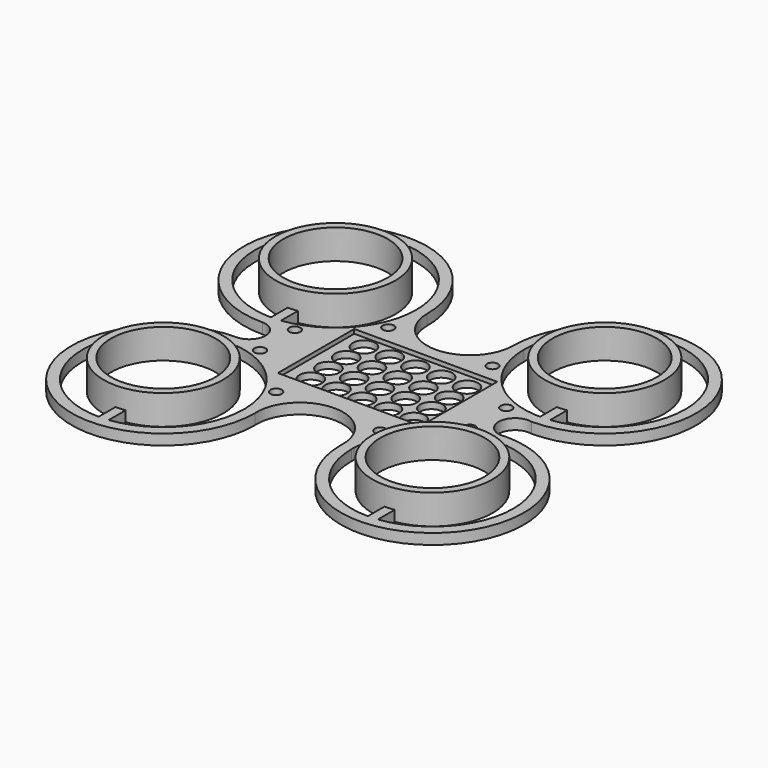
from build123d import *

# Parameters (mm, degrees)
F0_R     = 2.6543
F0_W     = 67.4656428301
F0_H     = 45.0660958886
F0_R_2   = 2.6574668283
F1_DEPTH = 5
F0_R_3   = 24.6634
F0_R_4   = 24.6579201523
F2_DEPTH = 4
F3_DEPTH = 10
F0_R_5   = 5.2850261196
F4_DEPTH = 3


# Not quite as in the source:
# - ends of sketch curves that miss each other by under 0.0002 mm in the source are joined


with BuildPart() as f1:
    # F0 (on Top) → F1 (new body)
    with BuildSketch(Plane.XY):
        with BuildLine():
            ThreePointArc((127, 43.18), (117.5777235877, 50.8), (127, 58.42))
            ThreePointArc((127, 58.42), (157.5328708116, 132.1328708116), (83.82, 101.6))
            ThreePointArc((83.82, 101.6), (63.4999991392, 81.2799974683), (43.18, 101.6))
            ThreePointArc((43.18, 101.6), (-30.5328708116, 132.1328708116), (0, 58.42))
            ThreePointArc((0, 58.42), (7.62, 50.8), (0, 43.18))
            ThreePointArc((0, 43.18), (-30.5328708116, -30.5328708116), (43.18, 0))
            ThreePointArc((43.18, 0), (63.5, 21.5136188611), (83.82, 0))
            ThreePointArc((83.82, 0), (157.5328708116, -30.5328708116), (127, 43.18))
        make_face()
        with BuildLine():
            ThreePointArc((131.5376346572, 63.7711767072), (129.2728652121, 63.5678546), (127, 63.5))
            ThreePointArc((127, 63.5), (125.778197507, 63.5195956079), (124.55765181, 63.5783622746))
            ThreePointArc((124.55765181, 63.5783622746), (112.565928289, 50.8), (124.55765181, 38.0216377254))
            ThreePointArc((124.55765181, 38.0216377254), (125.778197507, 38.0804043921), (127, 38.1))
            ThreePointArc((127, 38.1), (129.277372025, 38.0318757973), (131.5466, 37.8277468063))
            ThreePointArc((131.5466, 37.8277468063), (165.1, 0), (131.5466, -37.8277468063))
            ThreePointArc((131.5466, -37.8277468063), (129.277372025, -38.0318757973), (127, -38.1))
            ThreePointArc((127, -38.1), (100.0592316368, -26.9407683632), (88.9, 0))
            ThreePointArc((88.9, 0), (88.9063611266, 0.6961877498), (88.9254423823, 1.3921430304))
            ThreePointArc((88.9254423823, 1.3921430304), (63.5, 26.5870041852), (38.0745576177, 1.3921430304))
            ThreePointArc((38.0745576177, 1.3921430304), (38.0936388734, 0.6961877498), (38.1, 0))
            ThreePointArc((38.1, 0), (28.5029424797, -25.2822520753), (4.5466, -37.8277468063))
            ThreePointArc((4.5466, -37.8277468063), (2.277372025, -38.0318757973), (0, -38.1))
            ThreePointArc((0, -38.1), (-38.1, 0), (0, 38.1))
            ThreePointArc((0, 38.1), (12.7, 50.8), (0, 63.5))
            ThreePointArc((0, 63.5), (-38.1, 101.6), (0, 139.7))
            ThreePointArc((0, 139.7), (2.277372025, 139.6318757973), (4.5466, 139.4277468063))
            ThreePointArc((4.5466, 139.4277468063), (28.5029424797, 126.8822520753), (38.1, 101.6))
            ThreePointArc((38.1, 101.6), (63.5, 76.1999974683), (88.9, 101.6))
            ThreePointArc((88.9, 101.6), (99.7497914455, 128.2277324182), (126.1197445529, 139.6898300121))
            ThreePointArc((126.1197445529, 139.6898300121), (128.3955342395, 139.6744334716), (130.6663445529, 139.5231844341))
            ThreePointArc((130.6663445529, 139.5231844341), (165.097480066, 102.0381924437), (131.5376346572, 63.7711767072))
        make_face(mode=Mode.SUBTRACT)
        with BuildLine():
            ThreePointArc((0, 63.5), (2.277372025, 63.5681242027), (4.5466, 63.7722531937))
            Line((4.5466, 63.7722531937), (4.5466, 73.7106698774))
            ThreePointArc((4.5466, 73.7106698774), (2.2807411415, 73.4346928635), (0, 73.3425))
            Line((0, 73.3425), (0, 63.5))
        make_face()
        with BuildLine():
            Line((4.5466, 129.4893301226), (4.5466, 139.4277468063))
            ThreePointArc((4.5466, 139.4277468063), (2.277372025, 139.6318757973), (0, 139.7))
            Line((0, 139.7), (0, 129.8575))
            ThreePointArc((0, 129.8575), (2.2807411415, 129.7653071365), (4.5466, 129.4893301226))
        make_face()
        with BuildLine():
            Line((4.5466, 27.8240290125), (4.5466, 37.8277468063))
            ThreePointArc((4.5466, 37.8277468063), (2.277372025, 38.0318757973), (0, 38.1))
            Line((0, 38.1), (0, 28.1930516626))
            ThreePointArc((0, 28.1930516626), (2.2807755959, 28.1006445607), (4.5466, 27.8240290125))
        make_face()
        with BuildLine():
            ThreePointArc((0, -38.1), (2.277372025, -38.0318757973), (4.5466, -37.8277468063))
            Line((4.5466, -37.8277468063), (4.5466, -27.8240290125))
            ThreePointArc((4.5466, -27.8240290125), (2.2807755959, -28.1006445607), (0, -28.1930516626))
            Line((0, -28.1930516626), (0, -38.1))
        make_face()
        with BuildLine():
            ThreePointArc((124.55765181, 38.0216377254), (112.565928289, 50.8), (124.55765181, 63.5783622746))
            ThreePointArc((124.55765181, 63.5783622746), (99.2091429959, 75.5370326521), (88.9, 101.6))
            ThreePointArc((88.9, 101.6), (63.5, 76.1999974683), (38.1, 101.6))
            ThreePointArc((38.1, 101.6), (28.5029424797, 76.3177479247), (4.5466, 63.7722531937))
            ThreePointArc((4.5466, 63.7722531937), (2.277372025, 63.5681242027), (0, 63.5))
            ThreePointArc((0, 63.5), (12.7, 50.8), (0, 38.1))
            ThreePointArc((0, 38.1), (2.277372025, 38.0318757973), (4.5466, 37.8277468063))
            ThreePointArc((4.5466, 37.8277468063), (28.0362100648, 25.7988551142), (38.0745576177, 1.3921430304))
            ThreePointArc((38.0745576177, 1.3921430304), (63.5, 26.5870041852), (88.9254423823, 1.3921430304))
            ThreePointArc((88.9254423823, 1.3921430304), (99.6900222545, 26.566428355), (124.55765181, 38.0216377254))
        make_face()
        with Locations((38.6349633336, 18.2641260326)):
            Circle(F0_R, mode=Mode.SUBTRACT)
        with Locations((13.3296269923, 40.3755865991)):
            Circle(F0_R, mode=Mode.SUBTRACT)
        with Locations((88.0172178149, 18.018445)):
            Circle(F0_R, mode=Mode.SUBTRACT)
        with Locations((112.3398169875, 40.3755865991)):
            Circle(F0_R, mode=Mode.SUBTRACT)
        with Locations((13.0839459598, 61.2586289644)):
            Circle(F0_R, mode=Mode.SUBTRACT)
        with Locations((38.8806462288, 84.1071307659)):
            Circle(F0_R, mode=Mode.SUBTRACT)
        with Locations((63.501621415, 52.8839789331)):
            Rectangle(F0_W, F0_H, mode=Mode.SUBTRACT)
        with Locations((112.8311827779, 61.2586289644)):
            Circle(F0_R, mode=Mode.SUBTRACT)
        with Locations((87.9784226418, 84.1848701239)):
            Circle(F0_R_2, mode=Mode.SUBTRACT)
        with BuildLine():
            Line((130.6663445529, 129.6087763106), (130.6663445529, 139.5231844341))
            ThreePointArc((130.6663445529, 139.5231844341), (128.3955342395, 139.6744334716), (126.1197445529, 139.6898300121))
            Line((126.1197445529, 139.6898300121), (126.1197445529, 129.8340004808))
            ThreePointArc((126.1197445529, 129.8340004808), (128.3975888552, 129.8131242189), (130.6663445529, 129.6087763106))
        make_face()
        with BuildLine():
            Line((127, 73.3522809275), (127, 63.5))
            ThreePointArc((127, 63.5), (129.2728652121, 63.5678546), (131.5376346572, 63.7711767072))
            Line((131.5376346572, 63.7711767072), (131.5376346572, 73.7191193733))
            ThreePointArc((131.5376346572, 73.7191193733), (129.2762193835, 73.4441398974), (127, 73.3522809275))
        make_face()
        with BuildLine():
            ThreePointArc((131.5466, 37.8277468063), (129.277372025, 38.0318757973), (127, 38.1))
            Line((127, 38.1), (127, 28.3257955932))
            ThreePointArc((127, 28.3257955932), (129.2807048906, 28.2338286668), (131.5466, 27.958525076))
            Line((131.5466, 27.958525076), (131.5466, 37.8277468063))
        make_face()
        with BuildLine():
            ThreePointArc((127, -38.1), (129.277372025, -38.0318757973), (131.5466, -37.8277468063))
            Line((131.5466, -37.8277468063), (131.5466, -27.958525076))
            ThreePointArc((131.5466, -27.958525076), (129.2807048906, -28.2338286668), (127, -28.3257955932))
            Line((127, -28.3257955932), (127, -38.1))
        make_face()
    extrude(amount=F1_DEPTH)

    # F0 (on Top) → F2 (join)
    with BuildSketch(Plane.XY):
        with BuildLine():
            ThreePointArc((28.1930516626, 0), (21.4829082149, 18.2574044344), (4.5466, 27.8240290125))
            ThreePointArc((4.5466, 27.8240290125), (2.2807755959, 28.1006445607), (0, 28.1930516626))
            ThreePointArc((0, 28.1930516626), (-28.1930516626, 0), (0, -28.1930516626))
            ThreePointArc((0, -28.1930516626), (2.2807755959, -28.1006445607), (4.5466, -27.8240290125))
            ThreePointArc((4.5466, -27.8240290125), (21.4829082149, -18.2574044344), (28.1930516626, 0))
        make_face()
        Circle(F0_R_3, mode=Mode.SUBTRACT)
        with BuildLine():
            ThreePointArc((28.2575, 101.6), (21.5286071977, 119.9031521431), (4.5466, 129.4893301226))
            ThreePointArc((4.5466, 129.4893301226), (2.2807411415, 129.7653071365), (0, 129.8575))
            ThreePointArc((0, 129.8575), (-28.2575, 101.6), (0, 73.3425))
            ThreePointArc((0, 73.3425), (2.2807411415, 73.4346928635), (4.5466, 73.7106698774))
            ThreePointArc((4.5466, 73.7106698774), (21.5286071977, 83.2968478569), (28.2575, 101.6))
        make_face()
        with Locations((0, 101.6)):
            Circle(F0_R_3, mode=Mode.SUBTRACT)
        with BuildLine():
            ThreePointArc((126.1197445529, 129.8340004808), (98.7557107836, 101.1598188294), (127, 73.3522809275))
            ThreePointArc((127, 73.3522809275), (129.2762193835, 73.4441398974), (131.5376346572, 73.7191193733))
            ThreePointArc((131.5376346572, 73.7191193733), (148.5187297703, 83.3003305528), (155.2477190725, 101.6))
            ThreePointArc((155.2477190725, 101.6), (148.2308679021, 120.2328709791), (130.6663445529, 129.6087763106))
            ThreePointArc((130.6663445529, 129.6087763106), (128.3975888552, 129.8131242189), (126.1197445529, 129.8340004808))
        make_face()
        with Locations((127, 101.6)):
            Circle(F0_R_3, mode=Mode.SUBTRACT)
        with BuildLine():
            ThreePointArc((131.5466, 27.958525076), (129.2807048906, 28.2338286668), (127, 28.3257955932))
            ThreePointArc((127, 28.3257955932), (98.6742044068, 0), (127, -28.3257955932))
            ThreePointArc((127, -28.3257955932), (129.2807048906, -28.2338286668), (131.5466, -27.958525076))
            ThreePointArc((131.5466, -27.958525076), (148.5770336032, -18.3516298151), (155.3257955932, 0))
            ThreePointArc((155.3257955932, 0), (148.5770336032, 18.3516298151), (131.5466, 27.958525076))
        make_face()
        with Locations((127, 0)):
            Circle(F0_R_4, mode=Mode.SUBTRACT)
    extrude(amount=F2_DEPTH)

    # F3 (add): faces of the model
    f3_faces = [f1.faces().sort_by_distance(p)[0] for p in [
        (2.2162320404, 128.9686719497, 4),
        (129.2118381771, 74.2405078817, 4),
        (129.2161968149, 27.4352553985, 4),
        (27.3956317421, 0, 4),
    ]]
    extrude(f3_faces, amount=F3_DEPTH)

    # F0 (on Top) → F4 (join)
    with BuildSketch(Plane.XY):
        with Locations((63.501621415, 52.8839789331)):
            Rectangle(F0_W, F0_H)
        with Locations((39.8230690813, 37.1708342285)):
            Circle(F0_R_5, mode=Mode.SUBTRACT)
        with Locations((52.241603622, 36.8332513428)):
            Circle(F0_R_5, mode=Mode.SUBTRACT)
        with Locations((39.5965345407, 47.9224171143)):
            Circle(F0_R_5, mode=Mode.SUBTRACT)
        with Locations((52.0150690813, 47.5848342285)):
            Circle(F0_R_5, mode=Mode.SUBTRACT)
        with Locations((64.6601381626, 36.495668457)):
            Circle(F0_R_5, mode=Mode.SUBTRACT)
        with Locations((77.0786727033, 36.1580855713)):
            Circle(F0_R_5, mode=Mode.SUBTRACT)
        with Locations((89.4972072439, 35.8205026855)):
            Circle(F0_R_5, mode=Mode.SUBTRACT)
        with Locations((64.433603622, 47.2472513428)):
            Circle(F0_R_5, mode=Mode.SUBTRACT)
        with Locations((76.8521381626, 46.909668457)):
            Circle(F0_R_5, mode=Mode.SUBTRACT)
        with Locations((89.2706727033, 46.5720855713)):
            Circle(F0_R_5, mode=Mode.SUBTRACT)
        with Locations((39.37, 58.674)):
            Circle(F0_R_5, mode=Mode.SUBTRACT)
        with Locations((51.7885345407, 58.3364171143)):
            Circle(F0_R_5, mode=Mode.SUBTRACT)
        with Locations((39.1434654593, 69.4255828857)):
            Circle(F0_R_5, mode=Mode.SUBTRACT)
        with Locations((51.562, 69.088)):
            Circle(F0_R_5, mode=Mode.SUBTRACT)
        with Locations((64.2070690813, 57.9988342285)):
            Circle(F0_R_5, mode=Mode.SUBTRACT)
        with Locations((76.625603622, 57.6612513428)):
            Circle(F0_R_5, mode=Mode.SUBTRACT)
        with Locations((89.0441381626, 57.323668457)):
            Circle(F0_R_5, mode=Mode.SUBTRACT)
        with Locations((76.3990690813, 68.4128342285)):
            Circle(F0_R_5, mode=Mode.SUBTRACT)
        with Locations((63.9805345407, 68.7504171143)):
            Circle(F0_R_5, mode=Mode.SUBTRACT)
        with Locations((88.817603622, 68.0752513428)):
            Circle(F0_R_5, mode=Mode.SUBTRACT)
    extrude(amount=F4_DEPTH)


solid = f1.part
